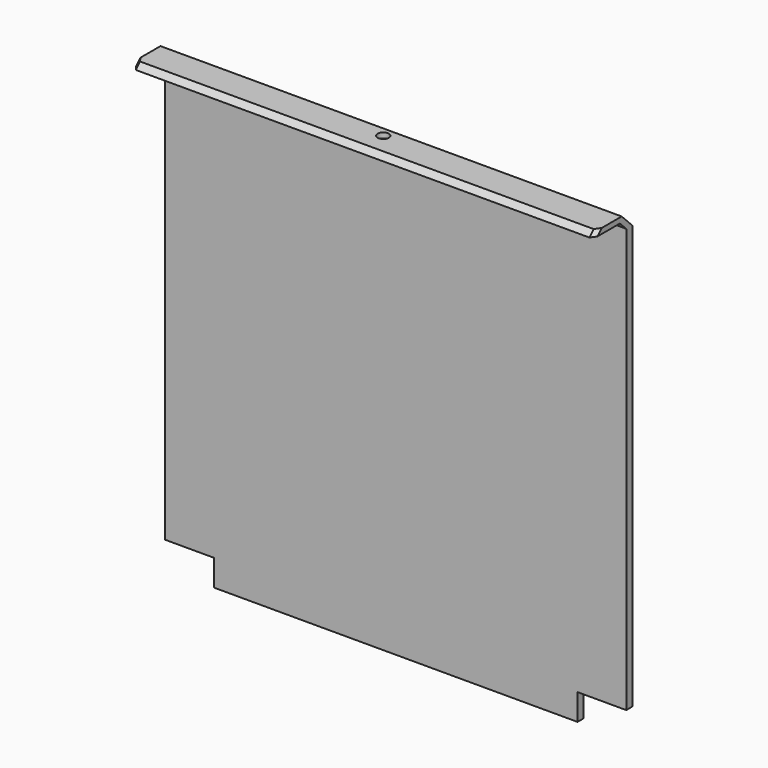
from build123d import *

# Parameters (mm, degrees)
F1_DEPTH   = 12.7
F1_FACE1_W = 781.05
F1_FACE1_H = 12.7
F4_SIZE    = 6.35
F6_D       = 19.05
F6_DEPTH   = 1524
F6_TIP     = 5.7231973962


with BuildPart() as f1:
    # F0 (on Front) → F1 (new body)
    with BuildSketch(Plane.XZ):
        Polygon((-307.975, -336.55), (-307.975, -381), (307.975, -381), (307.975, -336.55), (390.525, -336.55), (390.525, 381), (-390.525, 381), (-390.525, -336.55), align=None)
    extrude(amount=F1_DEPTH)

    # F3: sweep along a path in F2
    with BuildLine(Plane(origin=(-390.525, 0, 0), x_dir=(0, -1, 0), z_dir=(-1, 0, 0))) as f3_path:
        Line((6.35, 381), (24.3105122421, 398.9605122421))
        Line((24.3105122421, 398.9605122421), (78.2855122421, 398.9605122421))
    # F1_face1 (on face) → F3 (sweep)
    with BuildSketch(Plane(origin=(0, -6.35, 381), x_dir=(1, 0, 0), z_dir=(0, 0, 1))):
        Rectangle(F1_FACE1_W, F1_FACE1_H)
    sweep(path=f3_path.line, transition=Transition.RIGHT)

    # F4
    f4_edges = [f1.edges().sort_by_distance(p)[0] for p in [
        (-390.525, -78.285512, 398.960512),
        (390.525, -78.285512, 398.960512),
    ]]
    chamfer(f4_edges, length=F4_SIZE)

    # F6
    with Locations(Plane.XY.offset(403.4506403027)):
        with Locations((0, -38.8703841816)):
            Hole(F6_D / 2, depth=F6_DEPTH)
            with Locations((0, 0, -(F6_DEPTH + F6_TIP / 2))):  # 118° drill point
                Cone(0, F6_D / 2, F6_TIP, mode=Mode.SUBTRACT)


solid = f1.part
